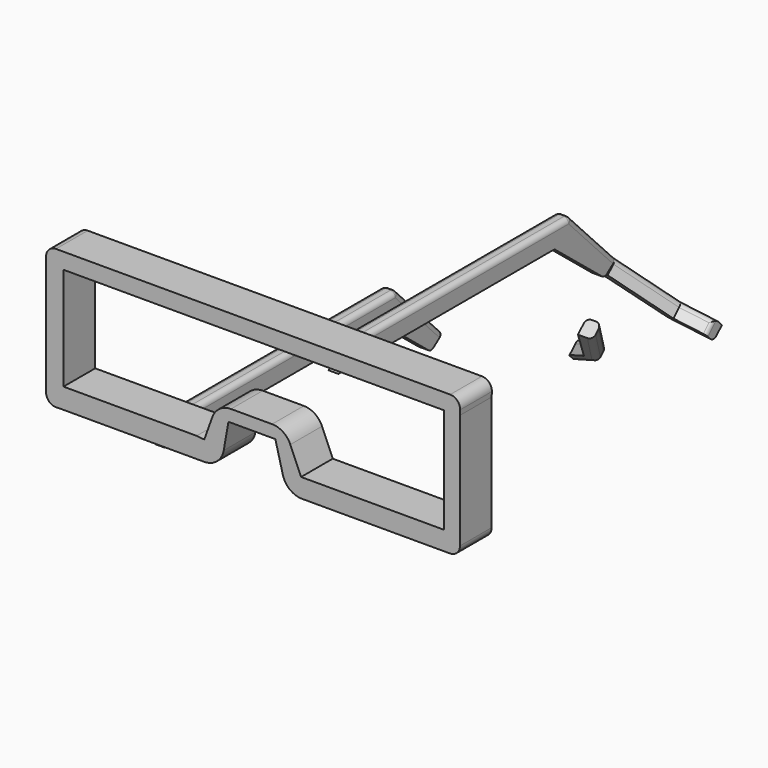
from build123d import *

# Parameters (mm, degrees)
F1_DEPTH = 10.16
F2_R     = 2.54
F3_R     = 5.08
F4_R     = 5.08
F6_DEPTH = 3.81
F9_DEPTH = 3.81
F10_R    = 1.27
F11_R    = 1.27


# Not quite as in the source:
# - the program builds the solid bodies; features that only make, move or delete a surface that nothing else refers to are left out


with BuildPart() as f1:
    # F0 (on Front) → F1 (new body)
    with BuildSketch(Plane.XZ):
        Polygon((44.9832062758, 34.2221398221), (-56.6167937242, 34.2221398221), (-58.7496179054, 34.2221398221), (-58.7496179054, 30.9259524707), (-58.7496179054, -1.6480916013), (-55.2584681449, -1.4541984311), (-13.9603054913, -1.4541984311), (-12.0213742499, 9.5977097372), (0, 9.5977097372), (2.9083968621, -1.6480916013), (47.3099252406, -1.6480916013), (47.3099252406, 30.3442754953), (47.4351830781, 34.2221398221), align=None)
        Polygon((-54.2900747594, 3.7809157825), (-54.2900747594, 30.1503807117), (43.2381642863, 30.1503807117), (43.2381642863, 3.1992365022), (6.5923654832, 3.1992365022), (2.5206109826, 12.700000461), (-14.929771112, 12.700000461), (-18.2134622678, 3.5870230732), (-20.1529909369, 3.7809157825), align=None, mode=Mode.SUBTRACT)
    extrude(amount=F1_DEPTH)

    # F2
    f2_edges = [f1.edges().sort_by_distance(p)[0] for p in [
        (-58.749618, -5.08, -1.648092),
        (47.309925, -5.08, -1.648092),
        (-58.749618, -5.08, 34.22214),
        (47.435183, -5.08, 34.22214),
    ]]
    fillet(f2_edges, radius=F2_R)

    # F3
    f3_edges = [f1.edges().sort_by_distance(p)[0] for p in [
        (-13.960305, -5.08, -1.454198),
        (2.908397, -5.08, -1.648092),
    ]]
    fillet(f3_edges, radius=F3_R)

    # F4
    f4_edges = [f1.edges().sort_by_distance(p)[0] for p in [
        (-14.929771, -5.08, 12.7),
        (2.520611, -5.08, 12.7),
    ]]
    fillet(f4_edges, radius=F4_R)


with BuildPart() as f6:
    # F5 (on Right) → F6 (new body)
    with BuildSketch(Plane.YZ):
        with BuildLine():
            add(Edge.make_bspline(
                [(9.2055564746, 21.8204872643), (9.2055564746, 24.3849344552), (5.2882982418, 24.3849344552)],
                knots=[0, 0, 0, 1.5707963268, 1.5707963268, 1.5707963268], degree=2, weights=[1, 0.7071067812, 1]))
            add(Edge.make_bspline(
                [(5.2882982418, 19.2560400733), (9.2055564746, 19.2560400733), (9.2055564746, 21.8204872643)],
                knots=[4.7123889804, 4.7123889804, 4.7123889804, 6.2831853072, 6.2831853072, 6.2831853072], degree=2, weights=[1, 0.7071067812, 1]))
            Line((5.2882982418, 19.2560400733), (74.4923436056, 19.2560400733))
            Line((74.4923436056, 19.2560400733), (90.4938727617, 6.3009290025))
            Line((90.4938727617, 6.3009290025), (94.2801907659, 9.1076251119))
            Line((94.2801907659, 9.1076251119), (79.5904770494, 24.3849344552))
            Line((79.5904770494, 24.3849344552), (5.2882982418, 24.3849344552))
        make_face()
    extrude(amount=F6_DEPTH)

    # F10
    f10_edges = [f6.edges().sort_by_distance(p)[0] for p in [
        (3.81, 42.439388, 24.384934),
        (1.905, 79.590477, 24.384934),
        (0, 42.439388, 24.384934),
        (0, 39.890321, 19.25604),
        (0, 82.493108, 12.778485),
        (0, 86.935334, 16.74628),
        (3.81, 86.935334, 16.74628),
        (1.905, 74.492344, 19.25604),
        (1.905, 90.493873, 6.300929),
    ]]
    fillet(f10_edges, radius=F10_R)


with BuildPart() as f9:
    # F8 (on face) → F9 (new body)
    with BuildSketch(Plane(origin=(0, 53.5383501487, 51.4791589847), x_dir=(-1, 0, 0), z_dir=(0, 0.7208332253, 0.6931085494))):
        Polygon((-8.8015166948, -76.8618048767), (0, -58.781327474), (-3.81, -58.781327474), (-11.4579806104, -75.3560811281), (-17.6276620477, -79.4318392873), (-17.6276620477, -82.6924517751), align=None)
    extrude(amount=-F9_DEPTH)

    # F11
    f11_edges = [f9.edges().sort_by_distance(p)[0] for p in [
        (4.400758, 97.799683, -0.049623),
        (4.400758, 100.546057, 2.591121),
        (13.214589, 106.086185, -8.667589),
        (7.63399, 100.024242, 3.133809),
        (14.542821, 107.180766, -4.308979),
        (17.627662, 107.22005, -7.098322),
    ]]
    fillet(f11_edges, radius=F11_R)


with BuildPart() as f12_1:
    # F12: copy of F9
    add(f9.part.moved(Location((0, 0, -15.875))))


with BuildPart() as f13_1:
    # F13: instance of F12_1
    add(f12_1.part.mirror(Plane.YZ))


with BuildPart() as f15_1:
    # F15: copy of F6
    add(f6.part.moved(Location((-44.45, 0, -31.115))))


solid = Compound([f1.part, f6.part, f9.part, f13_1.part, f15_1.part])
